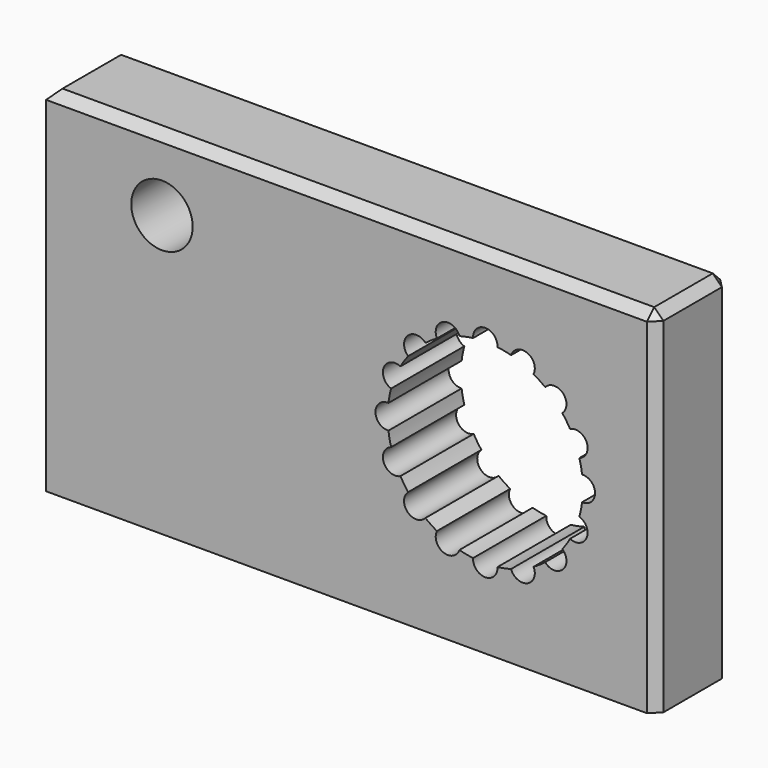
from build123d import *

# Parameters (mm, degrees)
F0_W     = 100
F0_H     = 58
F0_R     = 5.035
F1_DEPTH = 7.5
F2_SIZE  = 1.5


with BuildPart() as f1:
    # F0 (on Front) → F1 (new body, symmetric)
    with BuildSketch(Plane.XZ):
        Rectangle(F0_W, F0_H)
        with Locations((-31, 17)):
            Circle(F0_R, mode=Mode.SUBTRACT)
        with BuildLine():
            ThreePointArc((8.0972829663, 7.9192461182), (8.6964862032, 8.8891237283), (9.3632311248, 9.8138714275))
            ThreePointArc((9.3632311248, 9.8138714275), (9.2720779386, 12.7279220614), (12.1861285725, 12.6367688752))
            ThreePointArc((12.1861285725, 12.6367688752), (13.1108762717, 13.3035137968), (14.0807538818, 13.9027170337))
            ThreePointArc((14.0807538818, 13.9027170337), (15.1116982174, 16.6298315852), (17.7690471406, 15.4304581235))
            ThreePointArc((17.7690471406, 15.4304581235), (18.8785548477, 15.6925644865), (20.0039100722, 15.875))
            ThreePointArc((20.0039100722, 15.875), (22, 18), (23.9960899278, 15.875))
            ThreePointArc((23.9960899278, 15.875), (25.1214451523, 15.6925644865), (26.2309528594, 15.4304581235))
            ThreePointArc((26.2309528594, 15.4304581235), (28.8883017826, 16.6298315852), (29.9192461182, 13.9027170337))
            ThreePointArc((29.9192461182, 13.9027170337), (30.8891237283, 13.3035137968), (31.8138714275, 12.6367688752))
            ThreePointArc((31.8138714275, 12.6367688752), (34.7279220614, 12.7279220614), (34.6367688752, 9.8138714275))
            ThreePointArc((34.6367688752, 9.8138714275), (35.3035137968, 8.8891237283), (35.9027170337, 7.9192461182))
            ThreePointArc((35.9027170337, 7.9192461182), (38.6298315852, 6.8883017826), (37.4304581235, 4.2309528594))
            ThreePointArc((37.4304581235, 4.2309528594), (37.6925644865, 3.1214451523), (37.875, 1.9960899278))
            ThreePointArc((37.875, 1.9960899278), (40, 0), (37.875, -1.9960899278))
            ThreePointArc((37.875, -1.9960899278), (37.6925644865, -3.1214451523), (37.4304581235, -4.2309528594))
            ThreePointArc((37.4304581235, -4.2309528594), (38.6298315852, -6.8883017826), (35.9027170337, -7.9192461182))
            ThreePointArc((35.9027170337, -7.9192461182), (35.3035137968, -8.8891237283), (34.6367688752, -9.8138714275))
            ThreePointArc((34.6367688752, -9.8138714275), (34.7279220614, -12.7279220614), (31.8138714275, -12.6367688752))
            ThreePointArc((31.8138714275, -12.6367688752), (30.8891237283, -13.3035137968), (29.9192461182, -13.9027170337))
            ThreePointArc((29.9192461182, -13.9027170337), (28.8883017826, -16.6298315852), (26.2309528594, -15.4304581235))
            ThreePointArc((26.2309528594, -15.4304581235), (25.1214451523, -15.6925644865), (23.9960899278, -15.875))
            ThreePointArc((23.9960899278, -15.875), (22, -18), (20.0039100722, -15.875))
            ThreePointArc((20.0039100722, -15.875), (18.8785548477, -15.6925644865), (17.7690471406, -15.4304581235))
            ThreePointArc((17.7690471406, -15.4304581235), (15.1116982174, -16.6298315852), (14.0807538818, -13.9027170337))
            ThreePointArc((14.0807538818, -13.9027170337), (13.1108762717, -13.3035137968), (12.1861285725, -12.6367688752))
            ThreePointArc((12.1861285725, -12.6367688752), (9.2720779386, -12.7279220614), (9.3632311248, -9.8138714275))
            ThreePointArc((9.3632311248, -9.8138714275), (8.6964862032, -8.8891237283), (8.0972829663, -7.9192461182))
            ThreePointArc((8.0972829663, -7.9192461182), (5.3701684148, -6.8883017826), (6.5695418765, -4.2309528594))
            ThreePointArc((6.5695418765, -4.2309528594), (6.3074355135, -3.1214451523), (6.125, -1.9960899278))
            ThreePointArc((6.125, -1.9960899278), (4, 0), (6.125, 1.9960899278))
            ThreePointArc((6.125, 1.9960899278), (6.3074355135, 3.1214451523), (6.5695418765, 4.2309528594))
            ThreePointArc((6.5695418765, 4.2309528594), (5.3701684148, 6.8883017826), (8.0972829663, 7.9192461182))
        make_face(mode=Mode.SUBTRACT)
    extrude(amount=F1_DEPTH, both=True)

    # F2
    f2_edges = [f1.edges().sort_by_distance(p)[0] for p in [
        (50, 0, 29),
        (0, 7.5, 29),
        (0, -7.5, 29),
        (50, -7.5, 0),
        (50, 7.5, 0),
        (-50, 0, 29),
    ]]
    chamfer(f2_edges, length=F2_SIZE)


solid = f1.part
